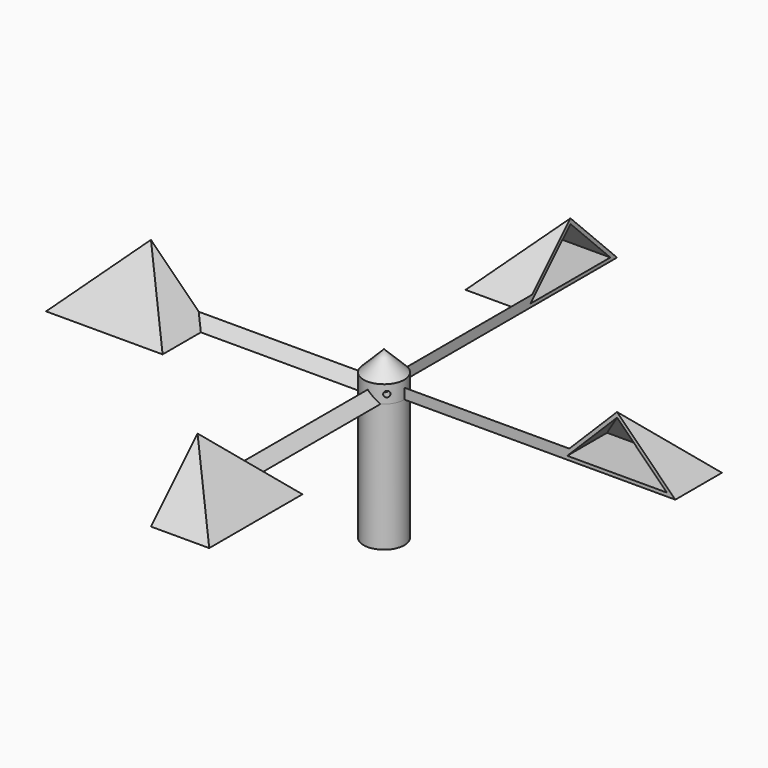
from build123d import *

# Parameters (mm, degrees)
F1_DEPTH    = 20
F2_T1_DEPTH = 122.8673195186
F2_T3_DEPTH = 142.8673195186
F3_T        = -1.2
F0_W        = 53
F0_H        = 3.6
F0_W_2      = 3.025
F4_DEPTH    = 5
F0_H_2      = 2.4
F6_T4_DEPTH = 84.4178503941
F6_S5_R     = 7
F6_T6_DEPTH = 44
F7_COUNT    = 4
F9_R        = 1
F10_DEPTH   = 141.4223562373


# Not quite as in the source:
# - a fillet or chamfer that OpenCascade refuses, or shapes differently, is made with other operations: its cross-section is extruded or revolved along the edge and cut away or added


with BuildPart() as f1:
    # F0 (on Front) → F1 (new body)
    with BuildSketch(Plane.XZ):
        Polygon((63.6, 3.6), (60, 0), (100, 0), (100, 20), (60, 20), (60, 3.6), align=None)
        Polygon((60, 3.6), (60, 0), (63.6, 3.6), align=None)
    extrude(amount=-F1_DEPTH)

    # F2: chamfer of 20 on 3 edges, made by hand

    # F2_s2 → F2_t1 (cut)
    with BuildSketch(Plane.XZ.offset(-71.4336597593)):
        Polygon((80, 20), (60, 0), (60, 20), align=None)
        Polygon((100, 0), (80, 20), (100, 20), align=None)
    extrude(amount=F2_T1_DEPTH, mode=Mode.SUBTRACT)

    # F2_s4 → F2_t3 (cut)
    with BuildSketch(Plane.YZ.offset(8.5663402407)):
        Polygon((0, 20), (20, 0), (20, 20), align=None)
    extrude(amount=F2_T3_DEPTH, mode=Mode.SUBTRACT)

    # F3
    f3_openings = [f1.faces().sort_by_distance(p)[0] for p in [
        (80, 0, 6.666667),
    ]]
    offset(amount=F3_T, openings=f3_openings)

    # F0 (on Front) → F4 (join)
    with BuildSketch(Plane.XZ):
        with Locations((33.5, 1.8)):
            Rectangle(F0_W, F0_H)
        Polygon((60, 3.6), (60, 0), (63.6, 3.6), align=None)
        with Locations((5.4875, 1.8)):
            Rectangle(F0_W_2, F0_H)
    extrude(amount=-F4_DEPTH)

    # F0 (on Front) → F5 (revolve)
    with BuildSketch(Plane.XZ):
        with Locations((5.4875, 4.8)):
            Rectangle(F0_W_2, F0_H_2)
        with Locations((5.4875, 1.8)):
            Rectangle(F0_W_2, F0_H)
        Polygon((0, 9.975), (3.975, 6), (7, 6), (0, 13), align=None)
    revolve(axis=Axis((0, 0, 3), (0, 0, 1)))

    # F6: chamfer of 5 on 1 edges, made by hand


with BuildPart() as f6_tool2:
    # F6_s3 → F6_t4 (new body)
    with BuildSketch(Plane.YZ.offset(76.4584149398)):
        Polygon((0, 3.6), (5, -1.4), (5, 3.6), align=None)
    extrude(amount=-F6_T4_DEPTH)

    # F6_s5 → F6_t6 (cut, symmetric)
    with BuildSketch(Plane.XY.offset(1.1)):
        Circle(F6_S5_R)
    extrude(amount=F6_T6_DEPTH, both=True, mode=Mode.SUBTRACT)

    split(bisect_by=Plane(origin=(30, 0, -30), x_dir=(0, 1, 0), z_dir=(-0.7071067812, 0, 0.7071067812)), keep=Keep.TOP)


with BuildPart() as f1_1:
    add(f1.part)

    # F6_t1: cut F6_tool2
    add(f6_tool2.part, mode=Mode.SUBTRACT)

    # F7: F1 ×4 about axis
    f7_axis = Axis((0, 0, 3), (0, 0, 1))


with BuildPart() as f1_2:
    add(f1_1.part)
    for i in range(1, F7_COUNT):
        add(f1_1.part.rotate(f7_axis, i * 360 / F7_COUNT))

    # F9 (on line) → F10 (cut, through all)
    with BuildSketch(Plane(origin=(0, 0, 0), x_dir=(-0.7071067812, -0.7071067812, 0), z_dir=(-0.7071067812, 0.7071067812, 0))):
        with Locations((0, 3)):
            Circle(F9_R)
    extrude(amount=-F10_DEPTH, mode=Mode.SUBTRACT)


with BuildPart() as f12:
    # F11 (on Front) → F12 (revolve)
    with BuildSketch(Plane.XZ):
        Polygon((3.975, 6), (0, 6), (0, -44), (7, -44), (7, 0), (3.975, 0), align=None)
    revolve(axis=Axis((0, 0, -19), (0, 0, 1)))


solid = Compound([f1_2.part, f12.part])
